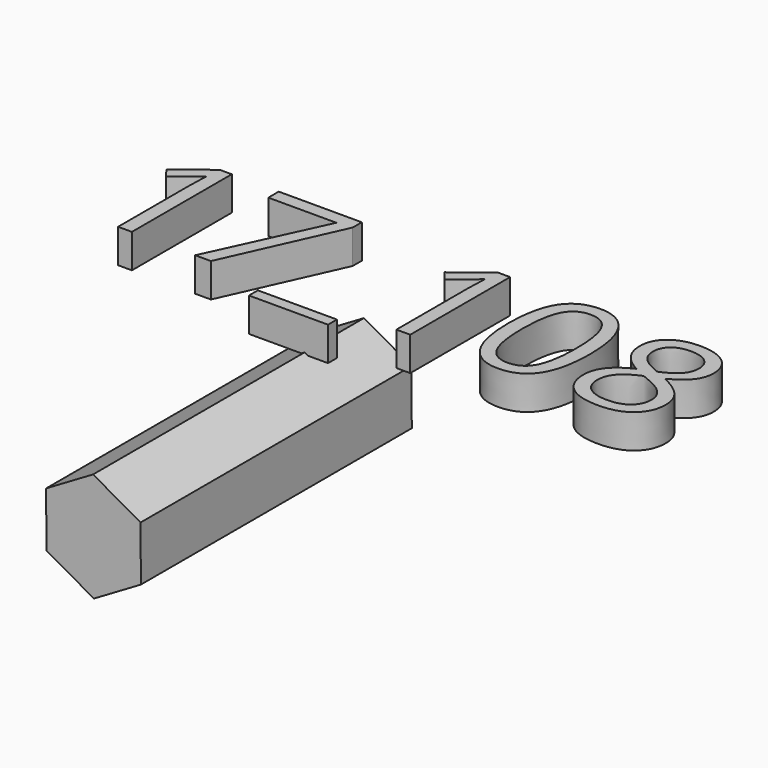
from build123d import *

# Parameters (mm, degrees)
F1_DEPTH     = 254
F3_TEXT_SIZE = 131.1757498317
F4_DEPTH     = 25.4


# Not quite as in the source:
# - Text() gives the source's letters only with a copy of the font that has no kerning and outlines rounded to 1/6400 em; it was checked with that copy


with BuildPart() as f1:
    # F0 (on Front) → F1 (new body)
    with BuildSketch(Plane.XZ):
        Polygon((50.3580224706, -6.062578898), (37.8737866033, -13.0223811462), (21.1506154734, -3.0292670153), (6.267503524, -9.6276837172), (-2.862703382, -44.525830938), (18.7291759003, -73.4227530345), (54.7840158773, -74.5584782782), (78.1517866615, -47.077782396), (71.5094416992, -13.0736098821), (66.985001961, -16.6354035112), (60.7326149984, -17.5376149613), (54.8667833294, -15.1927595155), (50.9592518126, -10.2291392966), align=None)
        Polygon((21.1506154734, -3.0292670153), (37.8737866033, -13.0223811462), (50.3580224706, -6.062578898), (50.0570403624, -3.9767523339), (51.1608646984, -1.2154530145), (39.2445645957, 4.9926719783), align=None)
        Polygon((0.5546615374, 9.2780709125), (21.1506154734, -3.0292670153), (39.2445645957, 4.9926719783), (51.1608646984, -1.2154530145), (52.4018958083, 1.8890793351), (57.3655160272, 5.7966108518), (63.6179029898, 6.698822302), (69.2269589248, 4.4566124846), (75.8461071349, 8.1467031785), (76.4993026007, 51.6162395619), (39.1801775348, 73.9166916206), (1.2078570031, 52.7476072959), align=None)
        Polygon((55.2403224163, -3.3407589565), (50.3580224706, -6.062578898), (50.9592518126, -10.2291392966), (54.8667833294, -15.1927595155), (60.7326149984, -17.5376149613), (66.985001961, -16.6354035112), (71.5094416992, -13.0736098821), (71.2360802368, -11.6741898913), align=None)
        Polygon((51.1608646984, -1.2154530145), (55.2403224163, -3.3407589565), (69.2269589248, 4.4566124846), (63.6179029898, 6.698822302), (57.3655160272, 5.7966108518), (52.4018958083, 1.8890793351), align=None)
        Polygon((69.2269589248, 4.4566124846), (55.2403224163, -3.3407589565), (71.2360802368, -11.6741898913), (71.5094416992, -13.0736098821), (71.9486221799, -12.7278719944), (74.2934776258, -6.8620403254), (73.3912661756, -0.6096533627), (69.4837346589, 4.3539668561), align=None)
    extrude(amount=F1_DEPTH)


with BuildPart() as f1b:
    # F0 (on Front) → F1, piece 2 (new body)
    with BuildSketch(Plane.XZ):
        Polygon((-40.3970259813, -80.4118015865), (-5.1259022566, -59.7042343517), (-5.4236196702, -18.8047615688), (-40.9924608084, 1.3871439794), (-76.2635845331, -19.3204232553), (-75.9658671195, -60.2198960383), align=None)
    extrude(amount=F1_DEPTH)

    # F3 (on Top) → F4 (join)
    with BuildSketch(Plane.XY):
        with Locations((-232.4185073376, -35.5799645185)):
            Text('17_108', F3_TEXT_SIZE, font='Open Sans', text_align=(TextAlign.LEFT, TextAlign.BOTTOM))
    extrude(amount=F4_DEPTH)


solid = f1b.part
